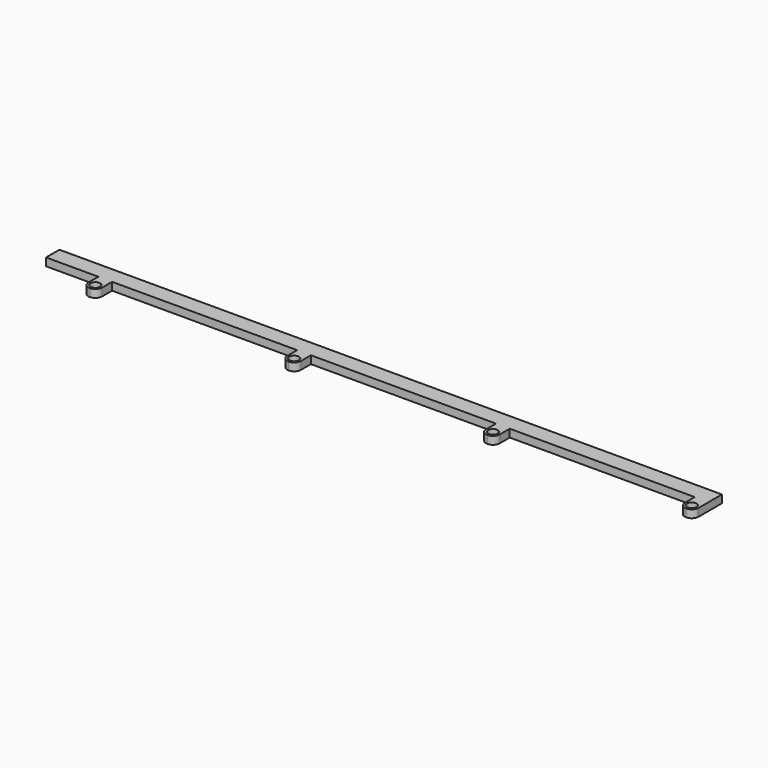
from build123d import *

# Parameters (mm, degrees)
F0_W     = 253.9
F0_H     = 6.4
F1_DEPTH = 3
F3_DEPTH = 3
F4_R     = 2.63999


# Not quite as in the source:
# - a fillet or chamfer is up to 0.001 mm smaller than in the source, because OpenCascade refuses the exact size


with BuildPart() as f1:
    # F0 (on Top) → F1 (new body)
    with BuildSketch(Plane.XY):
        Rectangle(F0_W, F0_H)
    extrude(amount=F1_DEPTH)

    # F2 (on Top) → F3 (join)
    with BuildSketch(Plane.XY):
        with BuildLine():
            Line((126.95, -10.59), (126.95, -3.2))
            Line((126.95, -3.2), (121.67, -3.2))
            Line((121.67, -3.2), (121.67, -7.95))
            Line((121.67, -7.95), (122.46, -7.95))
            ThreePointArc((122.46, -7.95), (124.31, -6.1), (126.16, -7.95))
            ThreePointArc((126.16, -7.95), (125.6181475452, -9.2581475452), (124.31, -9.8))
            Line((124.31, -9.8), (124.31, -10.59))
            Line((124.31, -10.59), (126.95, -10.59))
        make_face()
        with BuildLine():
            Line((122.46, -7.95), (121.67, -7.95))
            Line((121.67, -7.95), (121.67, -10.59))
            Line((121.67, -10.59), (124.31, -10.59))
            Line((124.31, -10.59), (124.31, -9.8))
            ThreePointArc((124.31, -9.8), (123.0018524548, -9.2581475452), (122.46, -7.95))
        make_face()
        Polygon((50.75, -10.59), (50.75, -3.2), (45.47, -3.2), (45.47, -7.95), (45.47, -10.59), align=None)
        with BuildLine():
            ThreePointArc((49.96, -7.95), (48.11, -9.8), (46.26, -7.95))
            ThreePointArc((46.26, -7.95), (48.11, -6.1), (49.96, -7.95))
        make_face(mode=Mode.SUBTRACT)
        Polygon((-101.65, -3.2), (-106.93, -3.2), (-106.93, -7.95), (-106.93, -10.59), (-101.65, -10.59), align=None)
        with BuildLine():
            ThreePointArc((-102.44, -7.95), (-104.29, -9.8), (-106.14, -7.95))
            ThreePointArc((-106.14, -7.95), (-104.29, -6.1), (-102.44, -7.95))
        make_face(mode=Mode.SUBTRACT)
        Polygon((-25.45, -3.2), (-30.73, -3.2), (-30.73, -7.95), (-30.73, -10.59), (-25.45, -10.59), align=None)
        with BuildLine():
            ThreePointArc((-26.24, -7.95), (-28.09, -9.8), (-29.94, -7.95))
            ThreePointArc((-29.94, -7.95), (-28.09, -6.1), (-26.24, -7.95))
        make_face(mode=Mode.SUBTRACT)
    extrude(amount=F3_DEPTH)

    # F4 (radius 2.64 in the source; OpenCascade refuses exactly that, so slightly less here)
    f4_edges = [f1.edges().sort_by_distance(p)[0] for p in [
        (45.47, -10.59, 1.5),
        (50.75, -10.59, 1.5),
        (121.67, -10.59, 1.5),
        (126.95, -10.59, 1.5),
        (-30.73, -10.59, 1.5),
        (-25.45, -10.59, 1.5),
        (-106.93, -10.59, 1.5),
        (-101.65, -10.59, 1.5),
    ]]
    fillet(f4_edges, radius=F4_R)


solid = f1.part
